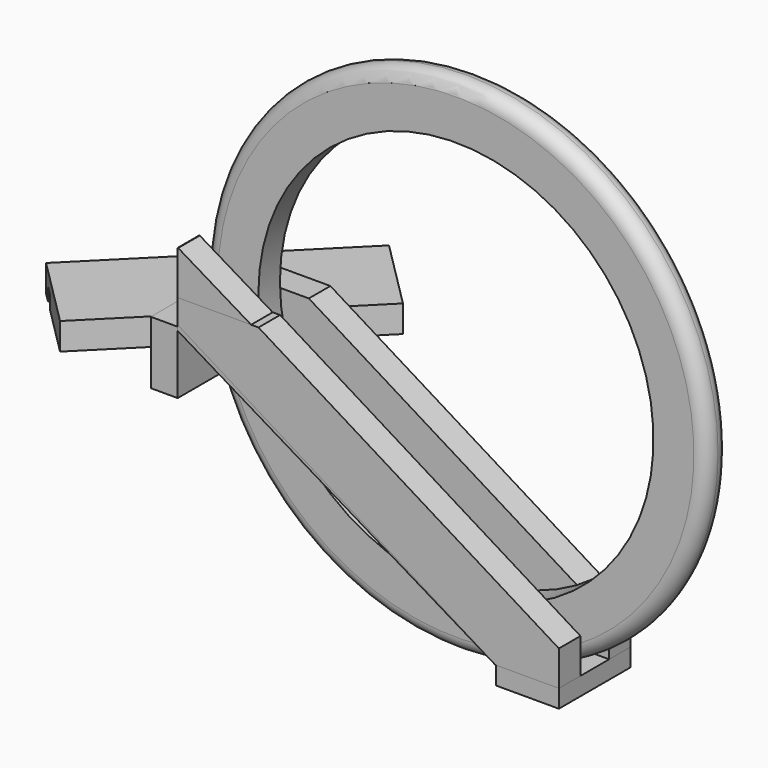
from build123d import *

# Parameters (mm, degrees)
F1_DEPTH  = 38.1
F2_W      = 88.9
F2_H      = 127
F3_DEPTH  = 25.4
F5_W      = 38.1
F5_H      = 88.9
F6_DEPTH  = 127
F8_R      = 355.6
F8_R_2    = 279.4
F9_DEPTH  = 38.1
F10_R     = 19.04999
F12_DEPTH = 38.1
F14_DEPTH = 19.05
F16_DEPTH = 38.1
F19_DEPTH = 38.1


# Not quite as in the source:
# - a fillet or chamfer is up to 0.001 mm smaller than in the source, because OpenCascade refuses the exact size


with BuildPart() as f1:
    # F0 (on Front) → F1 (new body)
    with BuildSketch(Plane.XZ):
        Polygon((0, 305.0617762964), (449.0947908261, 35.2184022785), (539.0602625189, 35.2184022785), (539.0602625189, 84.8754022785), (0.6535882854, 408.382769847), (0, 408.382769847), align=None)
    extrude(amount=F1_DEPTH)


with BuildPart() as f3:
    # F2 (on face) → F3 (new body)
    with BuildSketch(Plane(origin=(0, 0, 35.2184022785), x_dir=(1, 0, 0), z_dir=(0, 0, -1))):
        with Locations((494.6102625189, -25.4)):
            Rectangle(F2_W, F2_H)
    extrude(amount=F3_DEPTH)


with BuildPart() as f6:
    # F5 (on face) → F6 (new body)
    with BuildSketch(Plane.XZ.offset(38.1)):
        with Locations((-19.05, 265.6888514042)):
            Rectangle(F5_W, F5_H)
    extrude(amount=-F6_DEPTH)


with BuildPart() as f9:
    # F8 (on face) → F9 (new body)
    with BuildSketch(Plane(origin=(0, 0, 0), x_dir=(-1, 0, 0), z_dir=(0, 1, 0))):
        with Locations((-362.9855811596, 362.6356720924)):
            Circle(F8_R)
        with Locations((-362.9855811596, 362.6356720924)):
            Circle(F8_R_2, mode=Mode.SUBTRACT)
    extrude(amount=F9_DEPTH)

    # F10 (radius 19.05 in the source; OpenCascade refuses exactly that, so slightly less here)
    f10_edges = [f9.edges().sort_by_distance(p)[0] for p in [
        (718.585581, 0, 362.635672),
        (718.585581, 38.1, 362.635672),
    ]]
    fillet(f10_edges, radius=F10_R)


with BuildPart() as f12:
    # F11 (on face) → F12 (new body)
    with BuildSketch(Plane.XY.offset(310.1388514042)):
        Polygon((60.6828173318, 259.5248663003), (-208.7248663003, -9.8828173318), (-109.9420489686, -108.6656346635), (-38.1, -36.823585695), (-38.1, 88.9), (87.623585695, 88.9), (159.4656346635, 160.7420489686), align=None)
    extrude(amount=-F12_DEPTH)

    # F13 (on face) → F14 (cut)
    with BuildSketch(Plane(origin=(0, 0, 272.0388514042), x_dir=(1, 0, 0), z_dir=(0, 0, -1))):
        Polygon((-181.7840979371, 36.823585695), (-195.2544821187, 23.3532015134), (74.1532015134, -246.0544821187), (87.623585695, -232.5840979371), align=None)
    extrude(amount=-F14_DEPTH, mode=Mode.SUBTRACT)


with BuildPart() as f16:
    # F15 (on face) → F16 (new body)
    with BuildSketch(Plane(origin=(0, 88.9, 0), x_dir=(-1, 0, 0), z_dir=(0, 1, 0))):
        Polygon((-539.0602625189, 84.8846760996), (-539.0602625189, 35.2184022785), (-450.1602625189, 35.2184022785), (0, 312.3531075877), (0, 346.3848079563), (-114.2958221575, 346.3848079563), align=None)
    extrude(amount=-F16_DEPTH)


with BuildPart() as f19:
    # F18 (on face) → F19 (new body)
    with BuildSketch(Plane.XZ.offset(38.1)):
        Polygon((539.0602625189, 35.2184022785), (539.0602625189, 84.8846760996), (114.2958221575, 346.3848079563), (0, 346.3848079563), (0, 312.3531075877), (450.1602625189, 35.2184022785), align=None)
    extrude(amount=-F19_DEPTH)


solid = Compound([f1.part, f3.part, f6.part, f9.part, f12.part, f16.part, f19.part])
